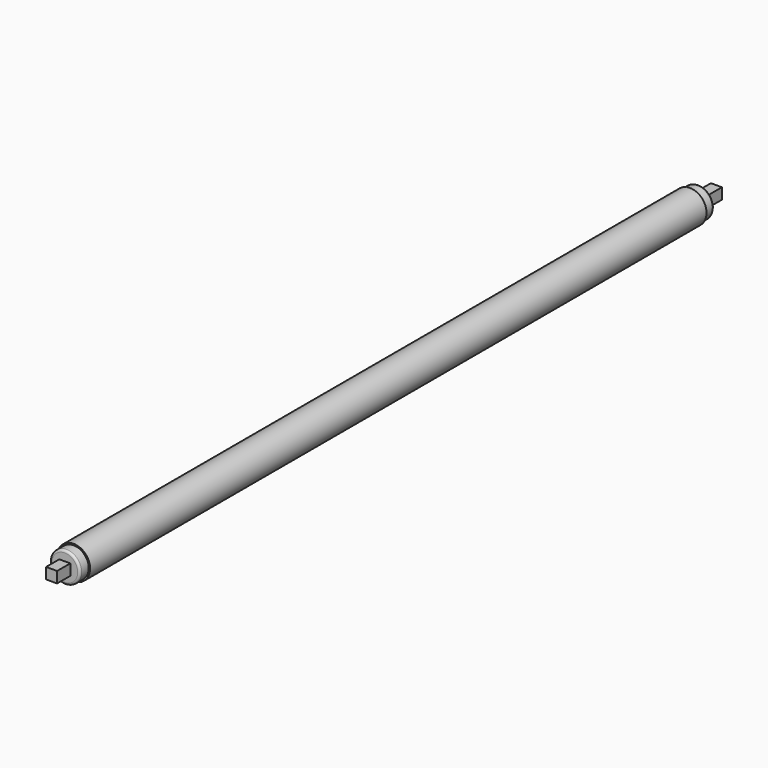
from build123d import *

# Parameters (mm, degrees)
F0_R     = 38.1
F1_DEPTH = 1778
F2_R     = 34.925
F3_DEPTH = 25.4
F4_R     = 34.925
F5_DEPTH = 25.4
F6_W     = 25.4
F6_H     = 25.4
F7_DEPTH = 38.1
F8_W     = 25.4
F8_H     = 25.4
F9_DEPTH = 38.1
F10_R    = 5.08
F11_R    = 5.08


# Not quite as in the source:
# - a pattern or mirror of a feature is missing from the dataset's text; its kind, count and spacing are read off the source's solid


with BuildPart() as f1:
    # F0 (on Front) → F1 (new body)
    with BuildSketch(Plane.XZ):
        Circle(F0_R)
    extrude(amount=F1_DEPTH)

    # F2 (on face) → F3 (join)
    with BuildSketch(Plane.XZ.offset(1778)):
        Circle(F2_R)
    extrude(amount=F3_DEPTH)

    # F4 (on face) → F5 (join)
    with BuildSketch(Plane(origin=(0, 0, 0), x_dir=(-1, 0, 0), z_dir=(0, 1, 0))):
        Circle(F4_R)
    extrude(amount=F5_DEPTH)

    # F6 (on face) → F7 (join)
    with BuildSketch(Plane.XZ.offset(1803.4)):
        Rectangle(F6_W, F6_H)
    f7 = extrude(amount=F7_DEPTH)

    # F7_copies: F7 across plane
    add(f7.mirror(Plane.ZX.offset(-882.65)))

    # F8 (on face) → F9 (join)
    with BuildSketch(Plane(origin=(0, 25.4, 0), x_dir=(-1, 0, 0), z_dir=(0, 1, 0))):
        Rectangle(F8_W, F8_H)
    extrude(amount=F9_DEPTH)

    # F10
    f10_edges = [f1.edges().sort_by_distance(p)[0] for p in [
        (34.925, 25.4, 0),
    ]]
    fillet(f10_edges, radius=F10_R)

    # F11
    f11_edges = [f1.edges().sort_by_distance(p)[0] for p in [
        (-34.925, -1803.4, 0),
    ]]
    fillet(f11_edges, radius=F11_R)


solid = f1.part
